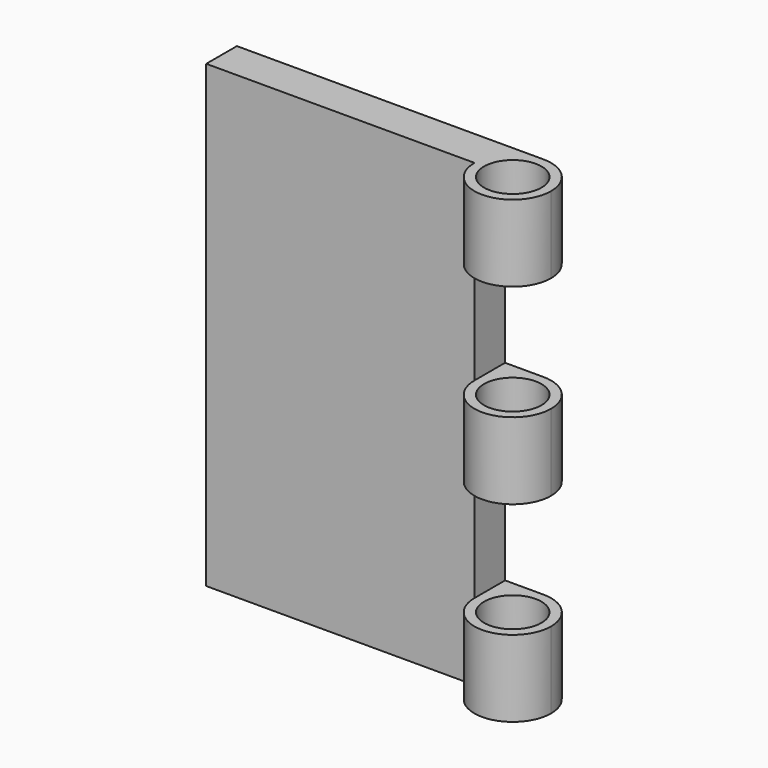
from build123d import *

# Parameters (mm, degrees)
F0_W     = 101.6
F0_H     = 152.4
F1_DEPTH = 12.7
F3_DEPTH = 152.4
F4_R     = 9.525
F5_DEPTH = 152.4
F7_W     = 50.8
F7_H     = 38.1
F8_DEPTH = 50.8


# Not quite as in the source:
# - a feature names something its author has since deleted; it is built from what else it names


with BuildPart() as f1:
    # F0 (on Front) → F1 (new body)
    with BuildSketch(Plane.XZ):
        with Locations((11.3006858155, 1.2977712616)):
            Rectangle(F0_W, F0_H)
    extrude(amount=F1_DEPTH)

    # F2 (on face) → F3 (join)
    with BuildSketch(Plane.XY.offset(77.4977712616)):
        with BuildLine():
            ThreePointArc((49.4006858155, -12.7), (62.1006858155, -25.4), (74.8006858155, -12.7))
            ThreePointArc((74.8006858155, -12.7), (71.0809419366, -3.7197438789), (62.1006858155, 0))
            Line((62.1006858155, 0), (62.1006858155, -12.7))
            Line((62.1006858155, -12.7), (49.4006858155, -12.7))
        make_face()
    extrude(amount=-F3_DEPTH)

    # F4 (on face) → F5 (cut, through all)
    with BuildSketch(Plane.XY.offset(77.4977712616)):
        with Locations((62.1006858155, -12.7)):
            Circle(F4_R)
    extrude(amount=-F5_DEPTH, mode=Mode.SUBTRACT)

    # F7 (on offset) → F8 (cut)
    with BuildSketch(Plane.XZ.offset(25.4)):
        with Locations((74.8006858155, 33.0477712616)):
            Rectangle(F7_W, F7_H)
        with Locations((74.8006858155, -30.4522287384)):
            Rectangle(F7_W, F7_H)
    extrude(amount=-F8_DEPTH, mode=Mode.SUBTRACT)


solid = f1.part
